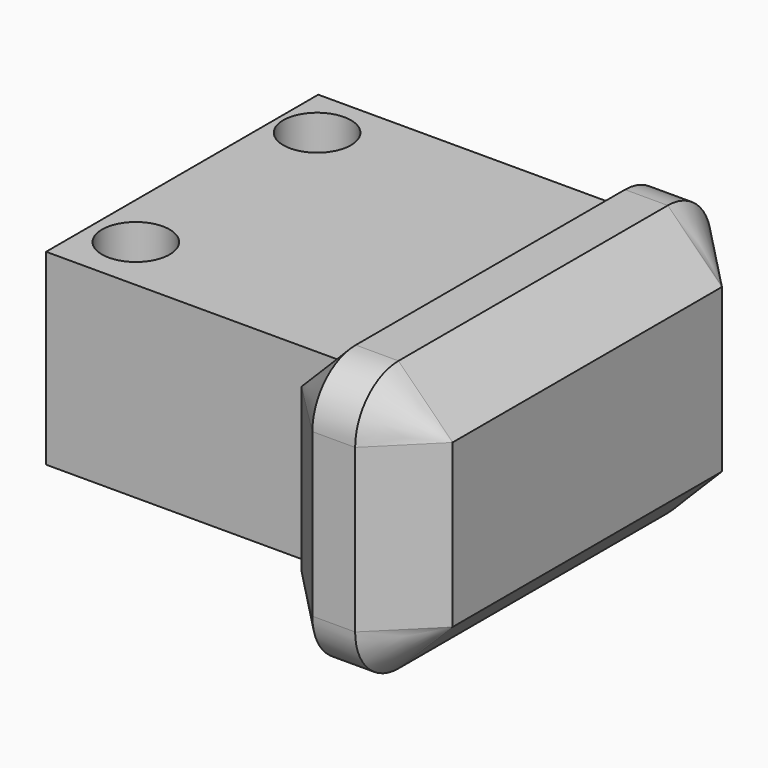
from build123d import *

# Parameters (mm, degrees)
F0_W          = 14.1733624041
F0_H          = 41.7313948274
F1_DEPTH      = 25.4
F2_R          = 5.08
F3_R          = 5.08
F4_R          = 5.08
F5_R          = 5.08
F6_W          = 31.9113396108
F6_H          = 17.5824901089
F7_DEPTH      = 12.7
F8_DEPTH      = 25.4
F10_D         = 6.35
F11_D         = 6.35
F12_T1_DEPTH  = 15.24
F12_T3_DEPTH  = 31.5713948274
F12_T6_ANGLE  = 90
F12_T8_ANGLE  = 90
F12_T10_ANGLE = 90
F12_T12_ANGLE = 90
F12_T14_ANGLE = 90
F12_T18_DEPTH = 31.5713948274
F12_T24_DEPTH = 31.5713948274
F12_T30_DEPTH = 31.5713948274
F12_T36_ANGLE = 90
F12_T42_ANGLE = 90
F12_T48_ANGLE = 90
F12_T54_DEPTH = 15.24
F12_T59_ANGLE = 90
F12_T65_ANGLE = 90
F12_T71_ANGLE = 90
F12_T77_DEPTH = 31.5713948274
F12_T83_DEPTH = 31.5713948274
F12_T89_DEPTH = 31.5713948274
F12_T93_ANGLE = 90


# Not quite as in the source:
# - a fillet or chamfer that OpenCascade refuses, or shapes differently, is made with other operations: its cross-section is extruded or revolved along the edge and cut away or added


with BuildPart() as f1:
    # F0 (on Top) → F1 (new body)
    with BuildSketch(Plane.XY):
        with Locations((-43.3002728969, -20.8656974137)):
            Rectangle(F0_W, F0_H)
    extrude(amount=F1_DEPTH)

    # F2
    f2_edges = [f1.edges().sort_by_distance(p)[0] for p in [
        (-43.300273, -41.731395, 25.4),
    ]]
    fillet(f2_edges, radius=F2_R)

    # F3
    f3_edges = [f1.edges().sort_by_distance(p)[0] for p in [
        (-43.300273, -41.731395, 0),
    ]]
    fillet(f3_edges, radius=F3_R)

    # F4
    f4_edges = [f1.edges().sort_by_distance(p)[0] for p in [
        (-43.300273, 0, 0),
    ]]
    fillet(f4_edges, radius=F4_R)

    # F5
    f5_edges = [f1.edges().sort_by_distance(p)[0] for p in [
        (-43.300273, 0, 25.4),
    ]]
    fillet(f5_edges, radius=F5_R)

    # F1_face (on face) + F6 (on face) → F7 (join)
    with BuildSketch(Plane(origin=(-50.3869540989, -20.8656974137, 12.7), x_dir=(0, -1, 0), z_dir=(-1, 0, 0))):
        with BuildLine():
            Line((-20.8656974137, 7.62), (-20.8656974137, -7.62))
            ThreePointArc((-20.8656974137, -7.62), (-19.3777998621, -11.2121024484), (-15.7856974137, -12.7))
            Line((-15.7856974137, -12.7), (15.7856974137, -12.7))
            ThreePointArc((15.7856974137, -12.7), (19.3777998621, -11.2121024484), (20.8656974137, -7.62))
            Line((20.8656974137, -7.62), (20.8656974137, 7.62))
            ThreePointArc((20.8656974137, 7.62), (19.3777998621, 11.2121024484), (15.7856974137, 12.7))
            Line((15.7856974137, 12.7), (-15.7856974137, 12.7))
            ThreePointArc((-15.7856974137, 12.7), (-19.3777998621, 11.2121024484), (-20.8656974137, 7.62))
        make_face()
    with BuildSketch(Plane(origin=(-50.3869540989, 0, 0), x_dir=(0, -1, 0), z_dir=(-1, 0, 0))):
        with Locations((18.8954193145, 13.6700686999)):
            Rectangle(F6_W, F6_H)
    extrude(amount=-F7_DEPTH)

    # F6 (on face) → F8 (join)
    with BuildSketch(Plane(origin=(-50.3869540989, 0, 0), x_dir=(0, -1, 0), z_dir=(-1, 0, 0))):
        with Locations((18.8954193145, 13.6700686999)):
            Rectangle(F6_W, F6_H)
    extrude(amount=F8_DEPTH)

    # F10 (through all)
    with Locations(Plane.XY.offset(22.4613137543)):
        with Locations((-71.6206654906, -29.537204653)):
            Hole(F10_D / 2)

    # F11 (through all)
    with Locations(Plane.XY.offset(22.4613137543)):
        with Locations((-72.0812156796, -7.7047413215)):
            Hole(F11_D / 2)

    # F12: chamfer of 5.08 on 4 edges, made by hand

    # F12_s2 → F12_t1 (cut)
    with BuildSketch(Plane.XY.offset(5.08)):
        Polygon((-36.2135916948, -36.6513948274), (-41.2935916948, -41.7313948274), (-36.2135916948, -41.7313948274), align=None)
        Polygon((-41.2935916948, 0), (-36.2135916948, -5.08), (-36.2135916948, 0), align=None)
        Polygon((-50.3869540989, -36.6513948274), (-45.3069540989, -41.7313948274), (-50.3869540989, -41.7313948274), align=None)
    extrude(amount=F12_T1_DEPTH, mode=Mode.SUBTRACT)

    # F12_s4 → F12_t3 (cut)
    with BuildSketch(Plane.XZ.offset(5.08)):
        Polygon((-36.2135916948, 20.32), (-41.2935916948, 25.4), (-36.2135916948, 25.4), align=None)
        Polygon((-36.2135916948, 5.08), (-41.2935916948, 0), (-36.2135916948, 0), align=None)
    extrude(amount=F12_T3_DEPTH, mode=Mode.SUBTRACT)

    # F12_s5 → F12_t6 (revolve, cut)
    with BuildSketch(Plane.XY.offset(20.32)):
        Polygon((-50.3869540989, -36.6513948274), (-45.3069540989, -41.7313948274), (-50.3869540989, -41.7313948274), align=None)
    revolve(axis=Axis((-50.3869540989, -36.6513948274, 20.32), (-1, 0, 0)), revolution_arc=F12_T6_ANGLE, mode=Mode.SUBTRACT)

    # F12_s7 → F12_t8 (revolve, cut)
    with BuildSketch(Plane.XY.offset(20.32)):
        Polygon((-36.2135916948, -36.6513948274), (-41.2935916948, -41.7313948274), (-36.2135916948, -41.7313948274), align=None)
    revolve(axis=Axis((-36.2135916948, -36.6513948274, 20.32), (-1, 0, 0)), revolution_arc=F12_T8_ANGLE, mode=Mode.SUBTRACT)

    # F12_s9 → F12_t10 (revolve, cut)
    with BuildSketch(Plane.XY.offset(20.32)):
        Polygon((-36.2135916948, -5.08), (-41.2935916948, 0), (-36.2135916948, 0), align=None)
    revolve(axis=Axis((-36.2135916948, -5.08, 20.32), (1, 0, 0)), revolution_arc=F12_T10_ANGLE, mode=Mode.SUBTRACT)

    # F12_s11 → F12_t12 (revolve, cut)
    with BuildSketch(Plane.XZ.offset(5.08)):
        Polygon((-41.2935916948, 0), (-36.2135916948, 5.08), (-36.2135916948, 0), align=None)
    revolve(axis=Axis((-36.2135916948, -5.08, 5.08), (1, 0, 0)), revolution_arc=F12_T12_ANGLE, mode=Mode.SUBTRACT)

    # F12_s13 → F12_t14 (revolve, cut)
    with BuildSketch(Plane.XY.offset(5.08)):
        Polygon((-36.2135916948, -36.6513948274), (-41.2935916948, -41.7313948274), (-36.2135916948, -41.7313948274), align=None)
    revolve(axis=Axis((-36.2135916948, -36.6513948274, 5.08), (1, 0, 0)), revolution_arc=F12_T14_ANGLE, mode=Mode.SUBTRACT)


with BuildPart() as f12_tool16:
    # F12_s17 → F12_t18 (new body)
    with BuildSketch(Plane.XZ.offset(5.08)):
        Polygon((-50.3869540989, 20.32), (-45.3069540989, 25.4), (-50.3869540989, 25.4), align=None)
    extrude(amount=F12_T18_DEPTH)

    split(bisect_by=Plane.XY.offset(22.4613137543), keep=Keep.TOP)

    split(bisect_by=Plane.XZ.offset(34.8510891199), keep=Keep.BOTTOM)


with BuildPart() as f1_1:
    add(f1.part)

    # F12_t15: cut F12_tool16
    add(f12_tool16.part, mode=Mode.SUBTRACT)


with BuildPart() as f12_tool22:
    # F12_s23 → F12_t24 (new body)
    with BuildSketch(Plane.XZ.offset(5.08)):
        Polygon((-50.3869540989, 20.32), (-45.3069540989, 25.4), (-50.3869540989, 25.4), align=None)
    extrude(amount=F12_T24_DEPTH)

    split(bisect_by=Plane.XY.offset(22.4613137543), keep=Keep.BOTTOM)

    split(bisect_by=Plane.XZ.offset(34.8510891199), keep=Keep.TOP)


with BuildPart() as f1_2:
    add(f1_1.part)

    # F12_t21: cut F12_tool22
    add(f12_tool22.part, mode=Mode.SUBTRACT)


with BuildPart() as f12_tool28:
    # F12_s29 → F12_t30 (new body)
    with BuildSketch(Plane.XZ.offset(5.08)):
        Polygon((-50.3869540989, 20.32), (-45.3069540989, 25.4), (-50.3869540989, 25.4), align=None)
    extrude(amount=F12_T30_DEPTH)

    split(bisect_by=Plane.XY.offset(22.4613137543), keep=Keep.TOP)

    split(bisect_by=Plane.XZ.offset(34.8510891199), keep=Keep.TOP)


with BuildPart() as f1_3:
    add(f1_2.part)

    # F12_t27: cut F12_tool28
    add(f12_tool28.part, mode=Mode.SUBTRACT)


with BuildPart() as f12_tool34:
    # F12_s35 → F12_t36 (revolve)
    with BuildSketch(Plane.XY.offset(20.32)):
        Polygon((-45.3069540989, 0), (-50.3869540989, -5.08), (-50.3869540989, 0), align=None)
    revolve(axis=Axis((-50.3869540989, -5.08, 20.32), (1, 0, 0)), revolution_arc=F12_T36_ANGLE)

    split(bisect_by=Plane.XZ.offset(2.9397495091), keep=Keep.BOTTOM)

    split(bisect_by=Plane.XY.offset(22.4613137543), keep=Keep.BOTTOM)


with BuildPart() as f1_4:
    add(f1_3.part)

    # F12_t33: cut F12_tool34
    add(f12_tool34.part, mode=Mode.SUBTRACT)


with BuildPart() as f12_tool40:
    # F12_s41 → F12_t42 (revolve)
    with BuildSketch(Plane.XY.offset(20.32)):
        Polygon((-45.3069540989, 0), (-50.3869540989, -5.08), (-50.3869540989, 0), align=None)
    revolve(axis=Axis((-50.3869540989, -5.08, 20.32), (1, 0, 0)), revolution_arc=F12_T42_ANGLE)

    split(bisect_by=Plane.XZ.offset(2.9397495091), keep=Keep.BOTTOM)

    split(bisect_by=Plane.XY.offset(22.4613137543), keep=Keep.TOP)


with BuildPart() as f1_5:
    add(f1_4.part)

    # F12_t39: cut F12_tool40
    add(f12_tool40.part, mode=Mode.SUBTRACT)


with BuildPart() as f12_tool46:
    # F12_s47 → F12_t48 (revolve)
    with BuildSketch(Plane.XY.offset(20.32)):
        Polygon((-45.3069540989, 0), (-50.3869540989, -5.08), (-50.3869540989, 0), align=None)
    revolve(axis=Axis((-50.3869540989, -5.08, 20.32), (1, 0, 0)), revolution_arc=F12_T48_ANGLE)

    split(bisect_by=Plane.XZ.offset(2.9397495091), keep=Keep.TOP)

    split(bisect_by=Plane.XY.offset(22.4613137543), keep=Keep.TOP)


with BuildPart() as f1_6:
    add(f1_5.part)

    # F12_t45: cut F12_tool46
    add(f12_tool46.part, mode=Mode.SUBTRACT)


with BuildPart() as f12_tool52:
    # F12_s53 → F12_t54 (new body)
    with BuildSketch(Plane.XY.offset(5.08)):
        Polygon((-45.3069540989, 0), (-50.3869540989, -5.08), (-50.3869540989, 0), align=None)
    extrude(amount=F12_T54_DEPTH)

    split(bisect_by=Plane.XZ.offset(2.9397495091), keep=Keep.BOTTOM)


with BuildPart() as f1_7:
    add(f1_6.part)

    # F12_t51: cut F12_tool52
    add(f12_tool52.part, mode=Mode.SUBTRACT)


with BuildPart() as f12_tool57:
    # F12_s58 → F12_t59 (revolve)
    with BuildSketch(Plane.XZ.offset(5.08)):
        Polygon((-45.3069540989, 0), (-50.3869540989, 5.08), (-50.3869540989, 0), align=None)
    revolve(axis=Axis((-50.3869540989, -5.08, 5.08), (1, 0, 0)), revolution_arc=F12_T59_ANGLE)

    split(bisect_by=Plane.XZ.offset(2.9397495091), keep=Keep.TOP)

    split(bisect_by=Plane.XY.offset(4.8788236454), keep=Keep.BOTTOM)


with BuildPart() as f1_8:
    add(f1_7.part)

    # F12_t56: cut F12_tool57
    add(f12_tool57.part, mode=Mode.SUBTRACT)


with BuildPart() as f12_tool63:
    # F12_s64 → F12_t65 (revolve)
    with BuildSketch(Plane.XZ.offset(5.08)):
        Polygon((-45.3069540989, 0), (-50.3869540989, 5.08), (-50.3869540989, 0), align=None)
    revolve(axis=Axis((-50.3869540989, -5.08, 5.08), (1, 0, 0)), revolution_arc=F12_T65_ANGLE)

    split(bisect_by=Plane.XZ.offset(2.9397495091), keep=Keep.BOTTOM)

    split(bisect_by=Plane.XY.offset(4.8788236454), keep=Keep.BOTTOM)


with BuildPart() as f1_9:
    add(f1_8.part)

    # F12_t62: cut F12_tool63
    add(f12_tool63.part, mode=Mode.SUBTRACT)


with BuildPart() as f12_tool69:
    # F12_s70 → F12_t71 (revolve)
    with BuildSketch(Plane.XZ.offset(5.08)):
        Polygon((-45.3069540989, 0), (-50.3869540989, 5.08), (-50.3869540989, 0), align=None)
    revolve(axis=Axis((-50.3869540989, -5.08, 5.08), (1, 0, 0)), revolution_arc=F12_T71_ANGLE)

    split(bisect_by=Plane.XZ.offset(2.9397495091), keep=Keep.BOTTOM)

    split(bisect_by=Plane.XY.offset(4.8788236454), keep=Keep.TOP)


with BuildPart() as f1_10:
    add(f1_9.part)

    # F12_t68: cut F12_tool69
    add(f12_tool69.part, mode=Mode.SUBTRACT)


with BuildPart() as f12_tool75:
    # F12_s76 → F12_t77 (new body)
    with BuildSketch(Plane.XZ.offset(5.08)):
        Polygon((-50.3869540989, 5.08), (-45.3069540989, 0), (-50.3869540989, 0), align=None)
    extrude(amount=F12_T77_DEPTH)

    split(bisect_by=Plane.XZ.offset(34.8510891199), keep=Keep.BOTTOM)

    split(bisect_by=Plane.XY.offset(4.8788236454), keep=Keep.BOTTOM)


with BuildPart() as f1_11:
    add(f1_10.part)

    # F12_t74: cut F12_tool75
    add(f12_tool75.part, mode=Mode.SUBTRACT)


with BuildPart() as f12_tool81:
    # F12_s82 → F12_t83 (new body)
    with BuildSketch(Plane.XZ.offset(5.08)):
        Polygon((-50.3869540989, 5.08), (-45.3069540989, 0), (-50.3869540989, 0), align=None)
    extrude(amount=F12_T83_DEPTH)

    split(bisect_by=Plane.XZ.offset(34.8510891199), keep=Keep.TOP)

    split(bisect_by=Plane.XY.offset(4.8788236454), keep=Keep.TOP)


with BuildPart() as f1_12:
    add(f1_11.part)

    # F12_t80: cut F12_tool81
    add(f12_tool81.part, mode=Mode.SUBTRACT)


with BuildPart() as f12_tool87:
    # F12_s88 → F12_t89 (new body)
    with BuildSketch(Plane.XZ.offset(5.08)):
        Polygon((-50.3869540989, 5.08), (-45.3069540989, 0), (-50.3869540989, 0), align=None)
    extrude(amount=F12_T89_DEPTH)

    split(bisect_by=Plane.XZ.offset(34.8510891199), keep=Keep.TOP)

    split(bisect_by=Plane.XY.offset(4.8788236454), keep=Keep.BOTTOM)


with BuildPart() as f1_13:
    add(f1_12.part)

    # F12_t86: cut F12_tool87
    add(f12_tool87.part, mode=Mode.SUBTRACT)

    # F12_s92 → F12_t93 (revolve, cut)
    with BuildSketch(Plane.XY.offset(5.08)):
        Polygon((-50.3869540989, -36.6513948274), (-45.3069540989, -41.7313948274), (-50.3869540989, -41.7313948274), align=None)
    revolve(axis=Axis((-50.3869540989, -36.6513948274, 5.08), (1, 0, 0)), revolution_arc=F12_T93_ANGLE, mode=Mode.SUBTRACT)


solid = f1_13.part
